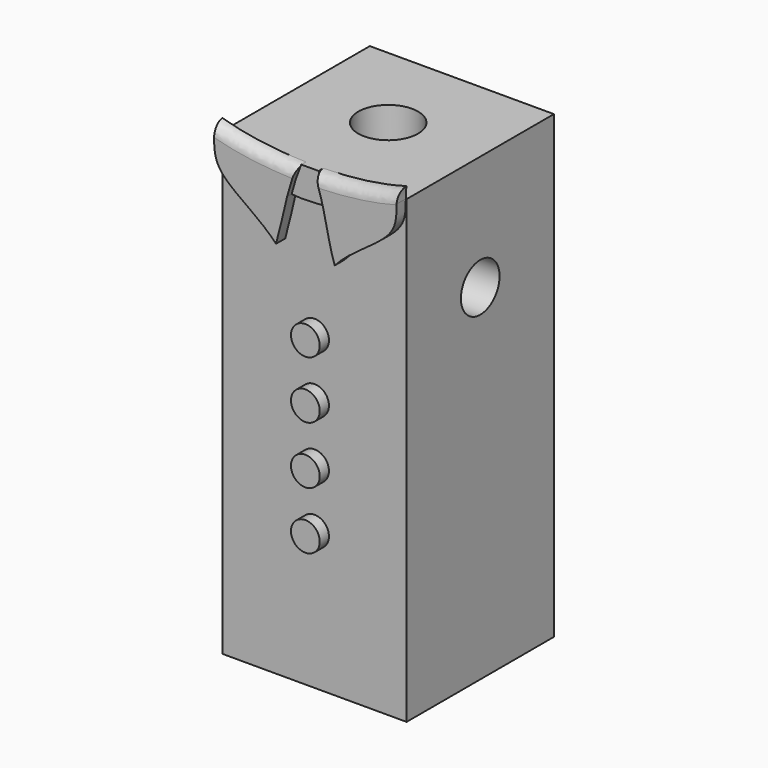
from build123d import *

# Parameters (mm, degrees)
F0_W      = 16
F0_H      = 40
F1_DEPTH  = 16
F2_R      = 2.6
F3_DEPTH  = 5
F4_R      = 2.1
F5_DEPTH  = 5
F6_R      = 2.1
F7_DEPTH  = 5
F8_R      = 2.1
F9_DEPTH  = 5
F10_R     = 2.1
F11_DEPTH = 5
F12_R     = 1.25
F13_DEPTH = 1
F14_R     = 1.25
F15_DEPTH = 1
F16_R     = 1.25
F17_DEPTH = 1
F18_R     = 1.25
F19_DEPTH = 1
F21_DEPTH = 1
F22_R     = 0.9999
F23_DEPTH = 0.5


# Not quite as in the source:
# - a fillet or chamfer is up to 0.001 mm smaller than in the source, because OpenCascade refuses the exact size


with BuildPart() as f1:
    # F0 (on Front) → F1 (new body)
    with BuildSketch(Plane.XZ):
        Rectangle(F0_W, F0_H)
    extrude(amount=F1_DEPTH)

    # F2 (on face) → F3 (cut)
    with BuildSketch(Plane.XY.offset(20)):
        with Locations((0, -8)):
            Circle(F2_R)
    extrude(amount=-F3_DEPTH, mode=Mode.SUBTRACT)

    # F4 (on face) → F5 (cut)
    with BuildSketch(Plane.YZ.offset(8)):
        with Locations((-8, 10)):
            Circle(F4_R)
    extrude(amount=-F5_DEPTH, mode=Mode.SUBTRACT)

    # F6 (on face) → F7 (cut)
    with BuildSketch(Plane(origin=(-8, 0, 0), x_dir=(0, -1, 0), z_dir=(-1, 0, 0))):
        with Locations((8, 10)):
            Circle(F6_R)
    extrude(amount=-F7_DEPTH, mode=Mode.SUBTRACT)

    # F8 (on face) → F9 (cut)
    with BuildSketch(Plane(origin=(0, 0, -20), x_dir=(1, 0, 0), z_dir=(0, 0, -1))):
        with Locations((4, 8)):
            Circle(F8_R)
    extrude(amount=-F9_DEPTH, mode=Mode.SUBTRACT)

    # F10 (on face) → F11 (cut)
    with BuildSketch(Plane(origin=(0, 0, -20), x_dir=(1, 0, 0), z_dir=(0, 0, -1))):
        with Locations((-4, 8)):
            Circle(F10_R)
    extrude(amount=-F11_DEPTH, mode=Mode.SUBTRACT)

    # F12 (on face) → F13 (join)
    with BuildSketch(Plane.XZ.offset(16)):
        with Locations((0, 7)):
            Circle(F12_R)
    extrude(amount=F13_DEPTH)

    # F14 (on face) → F15 (join)
    with BuildSketch(Plane.XZ.offset(16)):
        with Locations((0, 2)):
            Circle(F14_R)
    extrude(amount=F15_DEPTH)

    # F16 (on face) → F17 (join)
    with BuildSketch(Plane.XZ.offset(16)):
        with Locations((0, -3)):
            Circle(F16_R)
    extrude(amount=F17_DEPTH)

    # F18 (on face) → F19 (join)
    with BuildSketch(Plane.XZ.offset(16)):
        with Locations((0, -8)):
            Circle(F18_R)
    extrude(amount=F19_DEPTH)

    # F20 (on face) → F21 (join)
    with BuildSketch(Plane.XZ.offset(16)):
        with BuildLine():
            add(Edge.make_bspline(
                [(0.75, 20), (3.3594071533, 20.0532824127), (5.9301231166, 20.3851114773), (8, 21)],
                knots=[8.72055047, 8.72055047, 8.72055047, 8.72055047, 16, 16, 16, 16], degree=3))
            Line((0.75, 20), (7.9315101276, 20))
            add(Edge.make_bspline(
                [(8, 21), (7.936682093, 20.7032053334), (7.9331222274, 20.3617292136), (7.9315101276, 20)],
                knots=[0, 0, 0, 0, 0.1427572475, 0.1427572475, 0.1427572475, 0.1427572475], degree=3))
        make_face()
        with BuildLine():
            add(Edge.make_bspline(
                [(-8, 21), (-5.9479143878, 20.3884393869), (-3.3741827757, 20.0535723375), (-0.75, 20)],
                knots=[0, 0, 0, 0, 7.3266434187, 7.3266434187, 7.3266434187, 7.3266434187], degree=3))
            add(Edge.make_bspline(
                [(-8, 21), (-7.9392027192, 20.7034220667), (-7.9347343847, 20.3618566303), (-7.9314905291, 20)],
                knots=[0, 0, 0, 0, 0.1427309242, 0.1427309242, 0.1427309242, 0.1427309242], degree=3))
            Line((-7.9314905291, 20), (-0.75, 20))
        make_face()
        with BuildLine():
            Line((7.9315101276, 20), (0.75, 20))
            add(Edge.make_bspline(
                [(1.5735535475, 17.5164310059), (1.3638279631, 18.3834931797), (1.1151249806, 19.2296253371), (0.75, 20)],
                knots=[4.0589797926, 4.0589797926, 4.0589797926, 4.0589797926, 6.690552617, 6.690552617, 6.690552617, 6.690552617], degree=3))
            add(Edge.make_bspline(
                [(2.55, 13.5561273817), (2.1277926475, 14.7918965335), (1.8970376255, 16.1790605143), (1.5735535475, 17.5164310059)],
                knots=[0, 0, 0, 0, 4.0589797926, 4.0589797926, 4.0589797926, 4.0589797926], degree=3))
            add(Edge.make_bspline(
                [(7.9315101276, 20), (7.9285658859, 19.3393596044), (7.9402465057, 16.9450971177), (4.2150295862, 15.4292771095), (2.55, 13.5561273817)],
                knots=[0.1427572475, 0.1427572475, 0.1427572475, 0.1427572475, 0.4034804652, 1, 1, 1, 1], degree=3))
        make_face()
        with BuildLine():
            add(Edge.make_bspline(
                [(-1.5894267657, 17.4658260078), (-1.3661758267, 18.3343166755), (-1.104863981, 19.193579629), (-0.75, 20)],
                knots=[4.0525124649, 4.0525124649, 4.0525124649, 4.0525124649, 6.690552617, 6.690552617, 6.690552617, 6.690552617], degree=3))
            Line((-0.75, 20), (-7.9314905291, 20))
            add(Edge.make_bspline(
                [(-7.9314905291, 20), (-7.9255644562, 19.3389382799), (-7.9195168056, 16.9429139448), (-4.3261046571, 15.4424536286), (-2.55, 13.5561273817)],
                knots=[0.1427309242, 0.1427309242, 0.1427309242, 0.1427309242, 0.4034804652, 1, 1, 1, 1], degree=3))
            add(Edge.make_bspline(
                [(-2.55, 13.5561273817), (-2.185517021, 14.7757286924), (-1.9323810655, 16.1316653987), (-1.5894267657, 17.4658260078)],
                knots=[0, 0, 0, 0, 4.0525124649, 4.0525124649, 4.0525124649, 4.0525124649], degree=3))
        make_face()
    extrude(amount=F21_DEPTH)

    # F22 (radius 1 in the source; OpenCascade refuses exactly that, so slightly less here)
    f22_edges = [f1.edges().sort_by_distance(p)[0] for p in [
        (4.408175, -17, 20.266958),
        (-4.589536, -17, 20.290754),
    ]]
    fillet(f22_edges, radius=F22_R)

    # F20 (on face) → F23 (join)
    with BuildSketch(Plane.XZ.offset(16)):
        with BuildLine():
            Line((0.75, 20), (-0.75, 20))
            add(Edge.make_bspline(
                [(-0.75, 20), (-0.2507445203, 19.9898077667), (0.2503370769, 19.9897972051), (0.75, 20)],
                knots=[7.3266434187, 7.3266434187, 7.3266434187, 7.3266434187, 8.72055047, 8.72055047, 8.72055047, 8.72055047], degree=3))
        make_face()
        with BuildLine():
            add(Edge.make_bspline(
                [(-0.75, 20), (-0.2507445203, 19.9898077667), (0.2503370769, 19.9897972051), (0.75, 20)],
                knots=[7.3266434187, 7.3266434187, 7.3266434187, 7.3266434187, 8.72055047, 8.72055047, 8.72055047, 8.72055047], degree=3))
            add(Edge.make_bspline(
                [(-1.5894267657, 17.4658260078), (-1.3661758267, 18.3343166755), (-1.104863981, 19.193579629), (-0.75, 20)],
                knots=[4.0525124649, 4.0525124649, 4.0525124649, 4.0525124649, 6.690552617, 6.690552617, 6.690552617, 6.690552617], degree=3))
            add(Edge.make_bspline(
                [(-1.5894267657, 17.4658260078), (-0.646941675, 17.3500761834), (0.6084956384, 17.4665004575), (1.5735535475, 17.5164310059)],
                knots=[0, 0, 0, 0, 3.1633851058, 3.1633851058, 3.1633851058, 3.1633851058], degree=3))
            add(Edge.make_bspline(
                [(1.5735535475, 17.5164310059), (1.3638279631, 18.3834931797), (1.1151249806, 19.2296253371), (0.75, 20)],
                knots=[4.0589797926, 4.0589797926, 4.0589797926, 4.0589797926, 6.690552617, 6.690552617, 6.690552617, 6.690552617], degree=3))
        make_face()
    extrude(amount=F23_DEPTH)


solid = f1.part
